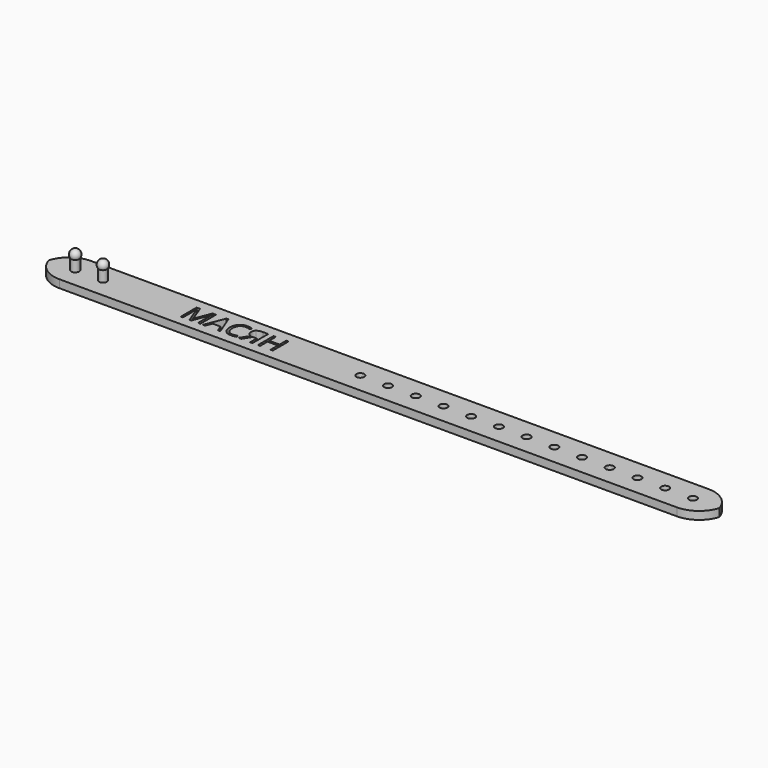
from build123d import *

# Parameters (mm, degrees)
F0_R     = 1
F1_DEPTH = 2
F2_R     = 1
F3_DEPTH = 3


# Not quite as in the source:
# - a feature names something its author has since deleted; it is built from what else it names


with BuildPart() as f1:
    # F0 (on Top) → F1 (new body)
    with BuildSketch(Plane.XY):
        with BuildLine():
            ThreePointArc((0.2917960675, 5), (2.8166998673, 1.3875139198), (7, 0))
            Line((7, 0), (163, 0))
            ThreePointArc((163, 0), (167.1833001327, 1.3875139198), (169.7082039325, 5))
            ThreePointArc((169.7082039325, 5), (167.1833001327, 8.6124860802), (163, 10))
            Line((163, 10), (7, 10))
            ThreePointArc((7, 10), (2.8166998673, 8.6124860802), (0.2917960675, 5))
        make_face()
        with BuildLine():
            Line((38.33984375, 2.5), (37.8754340278, 2.5))
            Line((37.8754340278, 2.5), (36.1935763889, 6.89453125))
            Line((36.1935763889, 6.89453125), (36.1664496528, 6.89453125))
            add(Edge.make_bspline(
                [(36.1664496528, 6.89453125), (36.2141927083, 6.3726128472), (36.2141927083, 5.6532118056)],
                knots=[0, 0, 0, 1, 1, 1], degree=2))
            Line((36.2141927083, 5.6532118056), (36.2141927083, 2.5))
            Line((36.2141927083, 2.5), (35.6814236111, 2.5))
            Line((35.6814236111, 2.5), (35.6814236111, 7.4576822917))
            Line((35.6814236111, 7.4576822917), (36.5494791667, 7.4576822917))
            Line((36.5494791667, 7.4576822917), (38.1195746528, 3.3680555556))
            Line((38.1195746528, 3.3680555556), (38.1467013889, 3.3680555556))
            Line((38.1467013889, 3.3680555556), (39.7298177083, 7.4576822917))
            Line((39.7298177083, 7.4576822917), (40.5913628472, 7.4576822917))
            Line((40.5913628472, 7.4576822917), (40.5913628472, 2.5))
            Line((40.5913628472, 2.5), (40.0151909722, 2.5))
            Line((40.0151909722, 2.5), (40.0151909722, 5.6944444444))
            add(Edge.make_bspline(
                [(40.0151909722, 5.6944444444), (40.0151909722, 6.2434895833), (40.0629340278, 6.8880208333)],
                knots=[0, 0, 0, 1, 1, 1], degree=2))
            Line((40.0629340278, 6.8880208333), (40.0358072917, 6.8880208333))
            Line((40.0358072917, 6.8880208333), (38.33984375, 2.5))
        make_face(mode=Mode.SUBTRACT)
        Polygon((45.6640625, 2.5), (45.0672743056, 2.5), (44.4498697917, 4.0766059028), (42.4631076389, 4.0766059028), (41.8532986111, 2.5), (41.26953125, 2.5), (43.2291666667, 7.4782986111), (43.7141927083, 7.4782986111), align=None, mode=Mode.SUBTRACT)
        with BuildLine():
            add(Edge.make_bspline(
                [(49.5941840278, 6.7491319444), (49.0310329861, 7.0128038194), (48.4678819444, 7.0128038194)],
                knots=[0, 0, 0, 1, 1, 1], degree=2))
            add(Edge.make_bspline(
                [(48.4678819444, 7.0128038194), (47.6508246528, 7.0128038194), (47.177734375, 6.4686414931)],
                knots=[0, 0, 0, 1, 1, 1], degree=2))
            add(Edge.make_bspline(
                [(47.177734375, 6.4686414931), (46.7046440972, 5.9244791667), (46.7046440972, 4.9782986111)],
                knots=[0, 0, 0, 1, 1, 1], degree=2))
            add(Edge.make_bspline(
                [(46.7046440972, 4.9782986111), (46.7046440972, 4.0060763889), (47.1609157986, 3.4749348958)],
                knots=[0, 0, 0, 1, 1, 1], degree=2))
            add(Edge.make_bspline(
                [(47.1609157986, 3.4749348958), (47.6171875, 2.9437934028), (48.4613715278, 2.9437934028)],
                knots=[0, 0, 0, 1, 1, 1], degree=2))
            add(Edge.make_bspline(
                [(48.4613715278, 2.9437934028), (48.9800347222, 2.9437934028), (49.6451822917, 3.1304253472)],
                knots=[0, 0, 0, 1, 1, 1], degree=2))
            Line((49.6451822917, 3.1304253472), (49.6451822917, 2.6258680556))
            add(Edge.make_bspline(
                [(49.6451822917, 2.6258680556), (49.1297743056, 2.431640625), (48.3734809028, 2.431640625)],
                knots=[0, 0, 0, 1, 1, 1], degree=2))
            add(Edge.make_bspline(
                [(48.3734809028, 2.431640625), (47.2786458333, 2.431640625), (46.6834852431, 3.0967881944)],
                knots=[0, 0, 0, 1, 1, 1], degree=2))
            add(Edge.make_bspline(
                [(46.6834852431, 3.0967881944), (46.0883246528, 3.7619357639), (46.0883246528, 4.9858940972)],
                knots=[0, 0, 0, 1, 1, 1], degree=2))
            add(Edge.make_bspline(
                [(46.0883246528, 4.9858940972), (46.0883246528, 5.751953125), (46.3747829861, 6.328125)],
                knots=[0, 0, 0, 1, 1, 1], degree=2))
            add(Edge.make_bspline(
                [(46.3747829861, 6.328125), (46.6612413194, 6.904296875), (47.2021484375, 7.2162543403)],
                knots=[0, 0, 0, 1, 1, 1], degree=2))
            add(Edge.make_bspline(
                [(47.2021484375, 7.2162543403), (47.7430555556, 7.5282118056), (48.4754774306, 7.5282118056)],
                knots=[0, 0, 0, 1, 1, 1], degree=2))
            add(Edge.make_bspline(
                [(48.4754774306, 7.5282118056), (49.2545572917, 7.5282118056), (49.8383246528, 7.2439236111)],
                knots=[0, 0, 0, 1, 1, 1], degree=2))
            Line((49.8383246528, 7.2439236111), (49.5941840278, 6.7491319444))
        make_face(mode=Mode.SUBTRACT)
        with BuildLine():
            Line((53.2063802083, 4.5681423611), (52.1983506944, 4.5681423611))
            Line((52.1983506944, 4.5681423611), (50.9006076389, 2.5))
            Line((50.9006076389, 2.5), (50.2180989583, 2.5))
            Line((50.2180989583, 2.5), (51.6091579861, 4.6668836806))
            add(Edge.make_bspline(
                [(51.6091579861, 4.6668836806), (51.0633680556, 4.8394097222), (50.8154296875, 5.1904296875)],
                knots=[0, 0, 0, 1, 1, 1], degree=2))
            add(Edge.make_bspline(
                [(50.8154296875, 5.1904296875), (50.5674913194, 5.5414496528), (50.5674913194, 6.0774739583)],
                knots=[0, 0, 0, 1, 1, 1], degree=2))
            add(Edge.make_bspline(
                [(50.5674913194, 6.0774739583), (50.5674913194, 6.7415364583), (51.0270182292, 7.099609375)],
                knots=[0, 0, 0, 1, 1, 1], degree=2))
            add(Edge.make_bspline(
                [(51.0270182292, 7.099609375), (51.4865451389, 7.4576822917), (52.4197048611, 7.4576822917)],
                knots=[0, 0, 0, 1, 1, 1], degree=2))
            Line((52.4197048611, 7.4576822917), (53.7825520833, 7.4576822917))
            Line((53.7825520833, 7.4576822917), (53.7825520833, 2.5))
            Line((53.7825520833, 2.5), (53.2063802083, 2.5))
            Line((53.2063802083, 2.5), (53.2063802083, 4.5681423611))
        make_face(mode=Mode.SUBTRACT)
        Polygon((58.9095052083, 7.4576822917), (58.9095052083, 2.5), (58.3333333333, 2.5), (58.3333333333, 4.8328993056), (55.7215711806, 4.8328993056), (55.7215711806, 2.5), (55.1453993056, 2.5), (55.1453993056, 7.4576822917), (55.7215711806, 7.4576822917), (55.7215711806, 5.3483072917), (58.3333333333, 5.3483072917), (58.3333333333, 7.4576822917), align=None, mode=Mode.SUBTRACT)
        with Locations((79.0238128991, 5)):
            Circle(F0_R, mode=Mode.SUBTRACT)
        with Locations((86.0238128991, 5)):
            Circle(F0_R, mode=Mode.SUBTRACT)
        with Locations((93.0238128991, 5)):
            Circle(F0_R, mode=Mode.SUBTRACT)
        with Locations((100.0238128991, 5)):
            Circle(F0_R, mode=Mode.SUBTRACT)
        with Locations((107.0238128991, 5)):
            Circle(F0_R, mode=Mode.SUBTRACT)
        with Locations((114.0238128991, 5)):
            Circle(F0_R, mode=Mode.SUBTRACT)
        with Locations((121.0238128991, 5)):
            Circle(F0_R, mode=Mode.SUBTRACT)
        with Locations((128.0238128991, 5)):
            Circle(F0_R, mode=Mode.SUBTRACT)
        with Locations((135.0238128991, 5)):
            Circle(F0_R, mode=Mode.SUBTRACT)
        with Locations((142.0238128991, 5)):
            Circle(F0_R, mode=Mode.SUBTRACT)
        with Locations((149.0238128991, 5)):
            Circle(F0_R, mode=Mode.SUBTRACT)
        with Locations((156.0238128991, 5)):
            Circle(F0_R, mode=Mode.SUBTRACT)
        with Locations((163.0238128991, 5)):
            Circle(F0_R, mode=Mode.SUBTRACT)
    extrude(amount=F1_DEPTH)

    # F2 (on face) → F3 (join)
    with BuildSketch(Plane.XY.offset(2)):
        with Locations((7, 5)):
            Circle(F2_R)
        with Locations((14, 5)):
            Circle(F2_R)
    extrude(amount=F3_DEPTH)


with BuildPart() as f1b:
    # F0 (on Top) → F1, piece 2 (new body)
    with BuildSketch(Plane.XY):
        with BuildLine():
            ThreePointArc((0, 3), (0.0733331419, 4.010587075), (0.2917960675, 5))
            ThreePointArc((0.2917960675, 5), (0.0733331419, 5.989412925), (0, 7))
            Line((0, 7), (0, 3))
        make_face()
    extrude(amount=F1_DEPTH)


with BuildPart() as f1c:
    # F0 (on Top) → F1, piece 3 (new body)
    with BuildSketch(Plane.XY):
        with BuildLine():
            ThreePointArc((170, 7), (169.9266668581, 5.989412925), (169.7082039325, 5))
            ThreePointArc((169.7082039325, 5), (169.9266668581, 4.010587075), (170, 3))
            Line((170, 3), (170, 7))
        make_face()
    extrude(amount=F1_DEPTH)


with BuildPart() as f7:
    # F6 (on offset) → F7 (revolve)
    with BuildSketch(Plane.XY.offset(5.5)):
        with BuildLine():
            Line((5.75, 5), (8.25, 5))
            ThreePointArc((8.25, 5), (7, 6.25), (5.75, 5))
        make_face()
    revolve(axis=Axis((7, 5, 5.5), (1, 0, 0)))


with BuildPart() as f9:
    # F8 (on offset) → F9 (revolve)
    with BuildSketch(Plane.XY.offset(5.5)):
        with BuildLine():
            Line((12.75, 5), (15.25, 5))
            ThreePointArc((15.25, 5), (14, 6.25), (12.75, 5))
        make_face()
    revolve(axis=Axis((14, 5, 5.5), (1, 0, 0)))


solid = Compound([f1.part, f7.part, f9.part])
